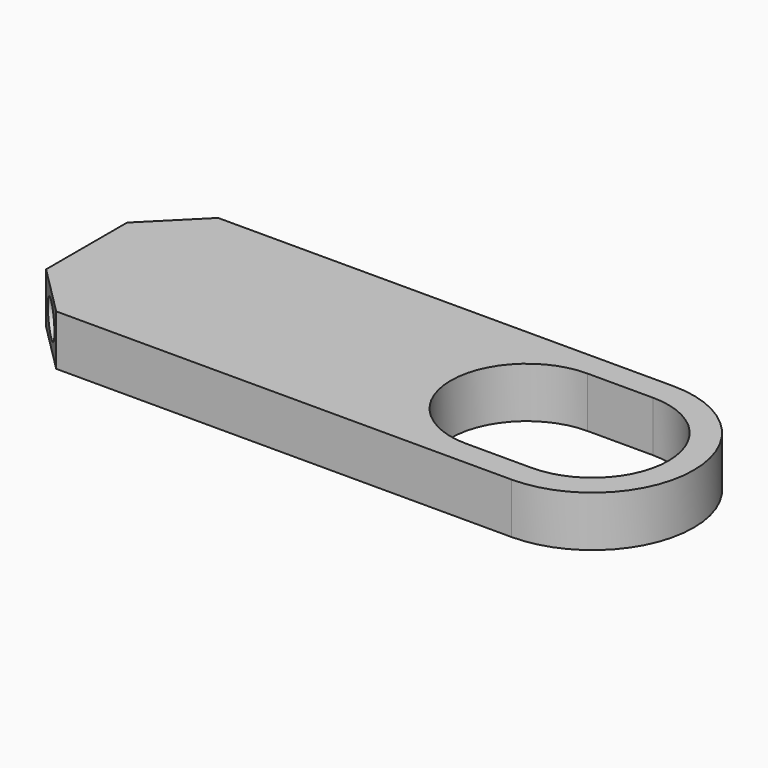
from build123d import *

# Parameters (mm, degrees)
F1_DEPTH    = 10
F2_R        = 3.25
F3_DEPTH    = 10
F4_T1_DEPTH = 61.4336597593


# Not quite as in the source:
# - a fillet or chamfer that OpenCascade refuses, or shapes differently, is made with other operations: its cross-section is extruded or revolved along the edge and cut away or added


with BuildPart() as f1:
    # F0 (on Top) → F1 (new body)
    with BuildSketch(Plane.XY):
        with BuildLine():
            Line((20, 20), (-80, 20))
            Line((-80, 20), (-80, -20))
            Line((-80, -20), (20, -20))
            ThreePointArc((20, -20), (40, 0), (20, 20))
        make_face()
        with BuildLine():
            ThreePointArc((20, 15), (35, 0), (20, -15))
            Line((20, -15), (7, -15))
            ThreePointArc((7, -15), (-8, 0), (7, 15))
            Line((7, 15), (20, 15))
        make_face(mode=Mode.SUBTRACT)
    extrude(amount=F1_DEPTH)

    # F2 (on face) → F3 (cut)
    with BuildSketch(Plane(origin=(-80, 0, 0), x_dir=(0, -1, 0), z_dir=(-1, 0, 0))):
        with Locations((-15, 5)):
            Circle(F2_R)
        with Locations((15, 5)):
            Circle(F2_R)
    extrude(amount=-F3_DEPTH, mode=Mode.SUBTRACT)

    # F4: chamfer of 10 on 2 edges, made by hand

    # F4_s2 → F4_t1 (cut)
    with BuildSketch(Plane.XY.offset(-25.7168298797)):
        Polygon((-70, 20), (-80, 10), (-80, 20), align=None)
        Polygon((-80, -10), (-70, -20), (-80, -20), align=None)
    extrude(amount=F4_T1_DEPTH, mode=Mode.SUBTRACT)


solid = f1.part
